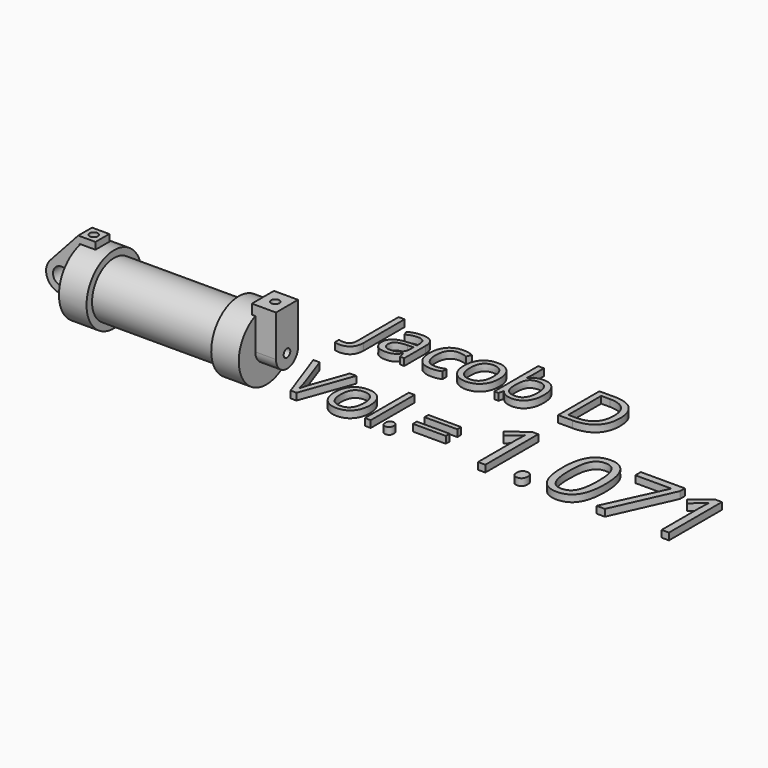
from build123d import *

# Parameters (mm, degrees)
F0_W          = 5.842
F0_H          = 12.7
F0_R          = 3.175
F2_DEPTH      = 3.175
F3_R          = 1.524
F4_DEPTH      = 7.62
F4_DEPTH_BACK = 1.27
F5_R          = 1.524
F6_DEPTH      = 10.414
F7_DEPTH      = 17.78
F5_TEXT_SIZE  = 26.6199310621
F8_TEXT_SIZE  = 34.1741730356
F9_DEPTH      = 2.54


# Not quite as in the source:
# - Text() gives the source's letters only with a copy of the font that has no kerning and outlines rounded to 1/6400 em; it was checked with that copy


with BuildPart() as f1:
    # F0 (on Front) → F1 (revolve)
    with BuildSketch(Plane.XZ):
        Polygon((5.842, 12.7), (5.842, 0), (66.294, 0), (66.294, 12.7), (56.134, 12.7), (56.134, 10.16), (10.16, 10.16), (10.16, 12.7), align=None)
        with Locations((2.921, 6.35)):
            Rectangle(F0_W, F0_H)
    revolve(axis=Axis((33.147, 0, 0), (-1, 0, 0)))

    # F3 (on face) → F4 (join, two sides)
    with BuildSketch(Plane.YZ.offset(66.294)) as f4_sk:
        with BuildLine():
            ThreePointArc((-5.08, 0), (0, -5.08), (5.08, 0))
            ThreePointArc((5.08, 0), (0, 5.08), (-5.08, 0))
        make_face()
        Circle(F3_R, mode=Mode.SUBTRACT)
        with BuildLine():
            ThreePointArc((-5.08, 0), (0, 5.08), (5.08, 0))
            Line((5.08, 0), (5.08, 15.24))
            Line((5.08, 15.24), (-5.08, 15.24))
            Line((-5.08, 15.24), (-5.08, 0))
        make_face()
    extrude(amount=F4_DEPTH)
    extrude(f4_sk.sketch, amount=-F4_DEPTH_BACK)

    # F5 (on face) → F6 (cut)
    with BuildSketch(Plane.XY.offset(15.24)):
        with Locations((69.5487681161, 0.0592393335)):
            Circle(F5_R)
    extrude(amount=-F6_DEPTH, mode=Mode.SUBTRACT)


with BuildPart() as f2:
    # F0 (on Front) → F2 (new body, symmetric)
    with BuildSketch(Plane.XZ):
        with BuildLine():
            Line((-0.9398, 0), (0, 0))
            Line((0, 0), (0, 12.7))
            Line((0, 12.7), (5.842, 12.7))
            Line((5.842, 12.7), (5.842, 15.24))
            Line((5.842, 15.24), (-0.508, 15.24))
            Line((-0.508, 15.24), (-10.8806298187, 3.8475430269))
            ThreePointArc((-10.8806298187, 3.8475430269), (-4.5919612295, 5.3297205562), (-0.9398, 0))
        make_face()
        with BuildLine():
            Line((5.842, 0), (0, 0))
            Line((0, 0), (-0.9398, 0))
            ThreePointArc((-0.9398, 0), (-3.1957909266, -4.5493385486), (-8.1826630726, -5.5069827884))
            Line((-8.1826630726, -5.5069827884), (5.842, -9.398))
            Line((5.842, -9.398), (5.842, 0))
        make_face()
        with BuildLine():
            ThreePointArc((-8.1826630726, -5.5069827884), (-3.1957909266, -4.5493385486), (-0.9398, 0))
            ThreePointArc((-0.9398, 0), (-4.5919612295, 5.3297205562), (-10.8806298187, 3.8475430269))
            ThreePointArc((-10.8806298187, 3.8475430269), (-12.1459778134, -1.5837270034), (-8.1826630726, -5.5069827884))
        make_face()
        with Locations((-6.6548, 0)):
            Circle(F0_R, mode=Mode.SUBTRACT)
    extrude(amount=F2_DEPTH, both=True)

    # F5 (on face) → F7 (cut)
    with BuildSketch(Plane.XY.offset(15.24)):
        with Locations((2.667, 0)):
            Circle(F5_R)
    extrude(amount=-F7_DEPTH, mode=Mode.SUBTRACT)


with BuildPart() as f9:
    # F5 (on face) + F8 (on face) → F9 (new body)
    with BuildSketch(Plane.XY.offset(15.24)):
        with Locations((103.8301438093, -8.071616292)):
            Text('Jacob D', F5_TEXT_SIZE, font='Open Sans', text_align=(TextAlign.LEFT, TextAlign.BOTTOM))
        with Locations((103.8301438093, -44.2747225364)):
            Text('Vol.=', F5_TEXT_SIZE, font='Open Sans', text_align=(TextAlign.LEFT, TextAlign.BOTTOM))
    with BuildSketch(Plane.XY.offset(15.24)):
        with Locations((171.3849753141, -45.355156064)):
            Text('1.071', F8_TEXT_SIZE, font='Open Sans', text_align=(TextAlign.LEFT, TextAlign.BOTTOM))
    extrude(amount=F9_DEPTH)


solid = Compound([f1.part, f2.part, f9.part])
